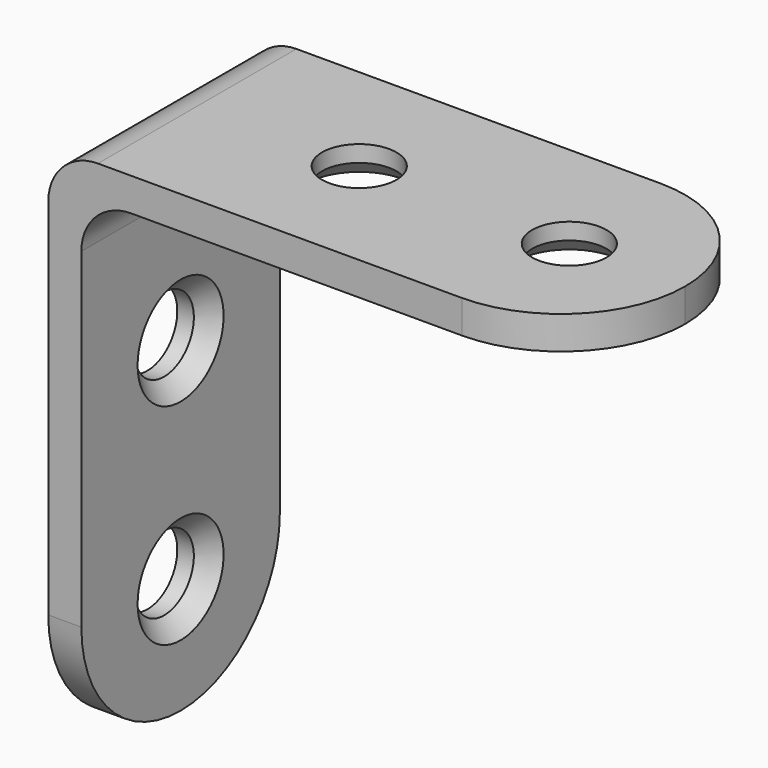
from build123d import *

# Parameters (mm, degrees)
F1_DEPTH             = 7.5
F2_R                 = 7.49999
F3_R                 = 3
F6_D                 = 4.5
F6_CSINK_D           = 6.5
F6_CSINK_ANGLE       = 90
F6_ON_F5_D           = 4.5
F6_ON_F5_CSINK_D     = 6.5
F6_ON_F5_CSINK_ANGLE = 90


# Not quite as in the source:
# - a fillet or chamfer is up to 0.001 mm smaller than in the source, because OpenCascade refuses the exact size


with BuildPart() as f1:
    # F0 (on Front) → F1 (new body, symmetric)
    with BuildSketch(Plane.XZ):
        Polygon((0, 0), (0, -32.5), (2, -32.5), (2, -2), (32.5, -2), (32.5, 0), align=None)
    extrude(amount=F1_DEPTH, both=True)

    # F2 (radius 7.5 in the source; OpenCascade refuses exactly that, so slightly less here)
    f2_edges = [f1.edges().sort_by_distance(p)[0] for p in [
        (32.5, -7.5, -1),
        (32.5, 7.5, -1),
        (1, -7.5, -32.5),
        (1, 7.5, -32.5),
    ]]
    fillet(f2_edges, radius=F2_R)

    # F3
    f3_edges = [f1.edges().sort_by_distance(p)[0] for p in [
        (2, 0, -2),
        (0, 0, 0),
    ]]
    fillet(f3_edges, radius=F3_R)

    # F6 (through all)
    with Locations(Plane(origin=(0, 0, -2), x_dir=(1, 0, 0), z_dir=(0, 0, -1))):
        with Locations((12.8, 0), (25.5, 0)):
            CounterSinkHole(F6_D / 2, F6_CSINK_D / 2, counter_sink_angle=F6_CSINK_ANGLE)

    # F6 on F5 (through all)
    with Locations(Plane.YZ.offset(2)):
        with Locations((0, -25.5), (0, -12.8)):
            CounterSinkHole(F6_ON_F5_D / 2, F6_ON_F5_CSINK_D / 2, counter_sink_angle=F6_ON_F5_CSINK_ANGLE)


solid = f1.part
